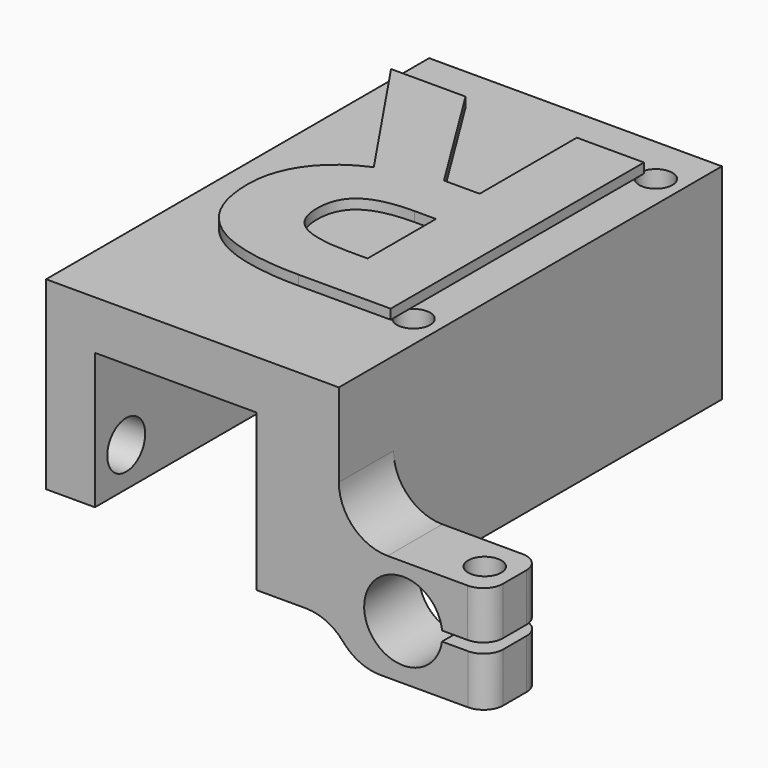
from build123d import *

# Parameters (mm, degrees)
F1_DEPTH      = 7
F2_DEPTH      = 42
F3_R          = 1.7
F3_R_2        = 11
F4_DEPTH      = 21.001
F5_R          = 4
F6_DEPTH      = 10
F7_DEPTH      = 21.001
F8_R          = 1.4
F9_DEPTH      = 11.027598684
F8_R_2        = 1.7
F10_DEPTH     = 4.9110969969
F11_R         = 5
F12_R         = 5
F13_R         = 5
F14_R         = 2
F15_R         = 2.2
F15_R_2       = 2.4255023423
F16_DEPTH     = 6
F17_TEXT_SIZE = 45.383431047
F18_DEPTH     = 1


# Not quite as in the source:
# - a feature names something its author has since deleted; it is built from what else it names
# - Text() gives the source's letters only with a copy of the font that has no kerning and outlines rounded to 1/6400 em; it was checked with that copy


with BuildPart() as f1:
    # F0 (on Front) → F1 (new body)
    with BuildSketch(Plane.XZ):
        Polygon((-18.6721007523, 29.8099789735), (-18.6721007523, 10.8925135386), (-13.6721007523, 10.8925135386), (-13.6721007523, 24.8099789735), (2.8778992477, 24.8099789735), (2.8778992477, 8.8099789735), (11.2880548998, 8.8099789735), (11.2880548998, 16.2656020473), (11.2880548998, 29.8099789735), align=None)
        Polygon((26.4763195603, 16.2417280634), (11.2880548998, 16.2656020473), (11.2880548998, 8.8099789735), (12.7033044869, 5.2860832236), (26.5053367778, 5.2860832236), (26.5053367778, 10.343908232), (19.8360510706, 10.343908232), (19.8360510706, 11.3388913612), (26.4763195603, 11.3388913612), align=None)
    extrude(amount=F1_DEPTH)

    # F0 (on Front) → F2 (join)
    with BuildSketch(Plane.XZ):
        Polygon((-18.6721007523, 29.8099789735), (-18.6721007523, 10.8925135386), (-13.6721007523, 10.8925135386), (-13.6721007523, 24.8099789735), (2.8778992477, 24.8099789735), (2.8778992477, 8.8099789735), (11.2880548998, 8.8099789735), (11.2880548998, 16.2656020473), (11.2880548998, 29.8099789735), align=None)
    extrude(amount=-F2_DEPTH)

    # F3 (on face) → F4 (cut, through all)
    with BuildSketch(Plane(origin=(0, 0, 8.8099789735), x_dir=(1, 0, 0), z_dir=(0, 0, -1))):
        with Locations((8.5280548998, -6)):
            Circle(F3_R)
        with Locations((8.5280548998, -37)):
            Circle(F3_R)
        with Locations((24.0280548998, -21.5)):
            Circle(F3_R_2)
    extrude(amount=-F4_DEPTH, mode=Mode.SUBTRACT)

    # F5 (on face) → F6 (cut)
    with BuildSketch(Plane.XZ.offset(7)):
        with Locations((17.8778992477, 10.8989789735)):
            Circle(F5_R)
    extrude(amount=-F6_DEPTH, mode=Mode.SUBTRACT)

    # F3 (on face) → F7 (cut, through all)
    with BuildSketch(Plane(origin=(0, 0, 8.8099789735), x_dir=(1, 0, 0), z_dir=(0, 0, -1))):
        with Locations((8.5280548998, -6)):
            Circle(F3_R)
        with Locations((8.5280548998, -37)):
            Circle(F3_R)
        with Locations((24.0280548998, -21.5)):
            Circle(F3_R_2)
    extrude(amount=-F7_DEPTH, mode=Mode.SUBTRACT)

    # F8 (on face) → F9 (cut, through all)
    with BuildSketch(Plane(origin=(0.0255952457, 0, 16.2833051745), x_dir=(0.9999987646, 0, -0.0015718685), z_dir=(0.0015718685, 0, 0.9999987646))):
        with Locations((23.4507569915, -3.5767070949)):
            Circle(F8_R)
    extrude(amount=-F9_DEPTH, mode=Mode.SUBTRACT)

    # F8 (on face) → F10 (cut, through all)
    with BuildSketch(Plane(origin=(0.0255952457, 0, 16.2833051745), x_dir=(0.9999987646, 0, -0.0015718685), z_dir=(0.0015718685, 0, 0.9999987646))):
        with Locations((23.4507569915, -3.5767070949)):
            Circle(F8_R_2)
        with Locations((23.4507569915, -3.5767070949)):
            Circle(F8_R, mode=Mode.SUBTRACT)
    extrude(amount=-F10_DEPTH, mode=Mode.SUBTRACT)

    # F11
    f11_edges = [f1.edges().sort_by_distance(p)[0] for p in [
        (11.288055, -3.5, 16.265602),
    ]]
    fillet(f11_edges, radius=F11_R)

    # F12
    f12_edges = [f1.edges().sort_by_distance(p)[0] for p in [
        (11.288055, -3.5, 8.809979),
    ]]
    fillet(f12_edges, radius=F12_R)

    # F13
    f13_edges = [f1.edges().sort_by_distance(p)[0] for p in [
        (12.703304, -3.5, 5.286083),
    ]]
    fillet(f13_edges, radius=F13_R)

    # F14
    f14_edges = [f1.edges().sort_by_distance(p)[0] for p in [
        (26.47632, -7, 13.79031),
        (26.505337, -7, 7.814996),
        (26.47632, 0, 13.79031),
        (26.505337, 0, 7.814996),
    ]]
    fillet(f14_edges, radius=F14_R)

    # F15 (on face) → F16 (cut)
    with BuildSketch(Plane(origin=(-18.6721007523, 0, 0), x_dir=(0, -1, 0), z_dir=(-1, 0, 0))):
        with Locations((-38, 14.8925135386)):
            Circle(F15_R)
        with Locations((3, 14.8925135386)):
            Circle(F15_R_2)
    extrude(amount=-F16_DEPTH, mode=Mode.SUBTRACT)

    # F17 (on face) → F18 (join)
    with BuildSketch(Plane.XY.offset(29.8099789735)):
        with Locations(Location((11.2880548998, 37.1265587479), (0, 0, 180))):
            Text('R', F17_TEXT_SIZE, font='Open Sans', font_style=FontStyle.BOLD, text_align=(TextAlign.LEFT, TextAlign.BOTTOM))
    extrude(amount=F18_DEPTH)


solid = f1.part
